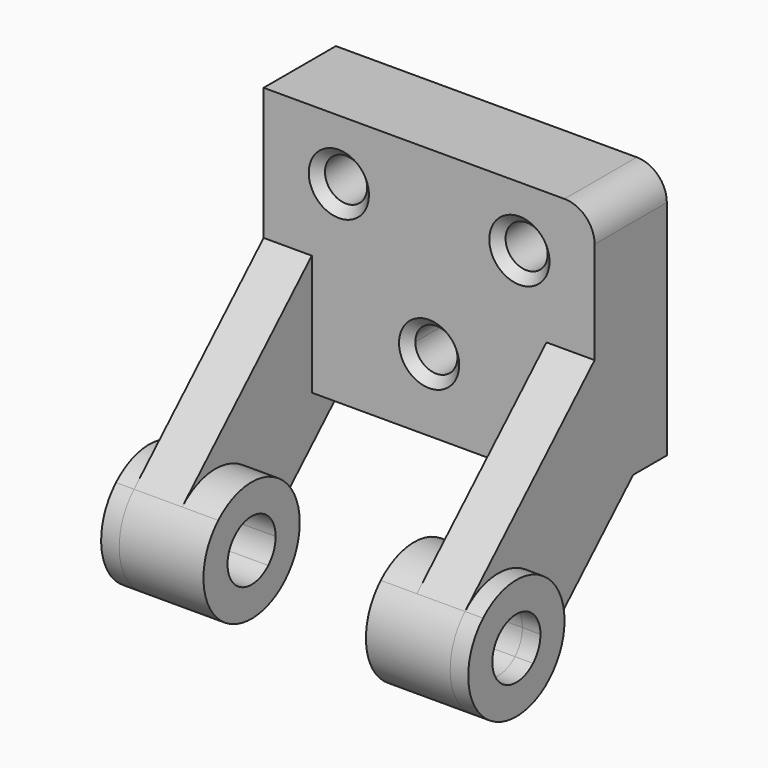
from build123d import *

# Parameters (mm, degrees)
F0_W           = 55
F0_H           = 42
F1_DEPTH       = 15
F3_DEPTH       = 8
F4_DEPTH       = 14
F4_DEPTH_BACK  = 3
F6_D           = 7
F6_CSINK_D     = 10
F6_CSINK_ANGLE = 90
F7_R           = 5


# Not quite as in the source:
# - a pattern or mirror of a feature is missing from the dataset's text; its kind, count and spacing are read off the source's solid


with BuildPart() as f1:
    # F0 (on Front) → F1 (new body)
    with BuildSketch(Plane.XZ):
        with Locations((0, -21)):
            Rectangle(F0_W, F0_H)
    extrude(amount=-F1_DEPTH)

    # F2 (on face) → F3 (join)
    with BuildSketch(Plane.YZ.offset(27.5)):
        with BuildLine():
            Line((0, -42), (0, -21.960586854))
            Line((0, -21.960586854), (-26.9221419573, -47.7830788612))
            ThreePointArc((-26.9221419573, -47.7830788612), (-16.0770814164, -45.8015919972), (-10, -55))
            ThreePointArc((-10, -55), (-10.8015919972, -58.9229185836), (-13.0778580427, -62.2169211388))
            Line((-13.0778580427, -62.2169211388), (8, -42))
            Line((8, -42), (0, -42))
        make_face()
    f3 = extrude(amount=-F3_DEPTH)

    # F3_copies: F3 across plane
    add(f3.mirror(Plane(origin=(0, 0, 0), x_dir=(0, 0, -1), z_dir=(-1, 0, 0))))

    # F2 (on face) → F4 (join, two sides)
    with BuildSketch(Plane.YZ.offset(27.5)) as f4_sk:
        with BuildLine():
            ThreePointArc((-10, -55), (-16.0770814164, -45.8015919972), (-26.9221419573, -47.7830788612))
            Line((-26.9221419573, -47.7830788612), (-23.4610709786, -51.3915394306))
            ThreePointArc((-23.4610709786, -51.3915394306), (-18.0385407082, -50.4007959986), (-15, -55))
            ThreePointArc((-15, -55), (-15.4007959986, -56.9614592918), (-16.5389290214, -58.6084605694))
            Line((-16.5389290214, -58.6084605694), (-13.0778580427, -62.2169211388))
            ThreePointArc((-13.0778580427, -62.2169211388), (-10.8015919972, -58.9229185836), (-10, -55))
        make_face()
        with BuildLine():
            Line((-23.4610709786, -51.3915394306), (-26.9221419573, -47.7830788612))
            ThreePointArc((-26.9221419573, -47.7830788612), (-27.2169211388, -61.9221419573), (-13.0778580427, -62.2169211388))
            Line((-13.0778580427, -62.2169211388), (-16.5389290214, -58.6084605694))
            ThreePointArc((-16.5389290214, -58.6084605694), (-23.6084605694, -58.4610709786), (-23.4610709786, -51.3915394306))
        make_face()
    f4 = extrude(amount=-F4_DEPTH) + extrude(f4_sk.sketch, amount=F4_DEPTH_BACK)

    # F4_copies: F4 across plane
    add(f4.mirror(Plane(origin=(0, 0, 0), x_dir=(0, 0, -1), z_dir=(-1, 0, 0))))

    # F6 (through all)
    with Locations(Plane.XZ):
        with Locations((-15, -10), (0, -30)):
            f6 = CounterSinkHole(F6_D / 2, F6_CSINK_D / 2, counter_sink_angle=F6_CSINK_ANGLE)

    # F6_copies: F6 across plane
    add(f6.mirror(Plane(origin=(0, 0, 0), x_dir=(0, 0, 1), z_dir=(1, 0, 0))), mode=Mode.SUBTRACT)

    # F7
    f7_edges = [f1.edges().sort_by_distance(p)[0] for p in [
        (27.5, 7.5, 0),
    ]]
    fillet(f7_edges, radius=F7_R)


solid = f1.part
